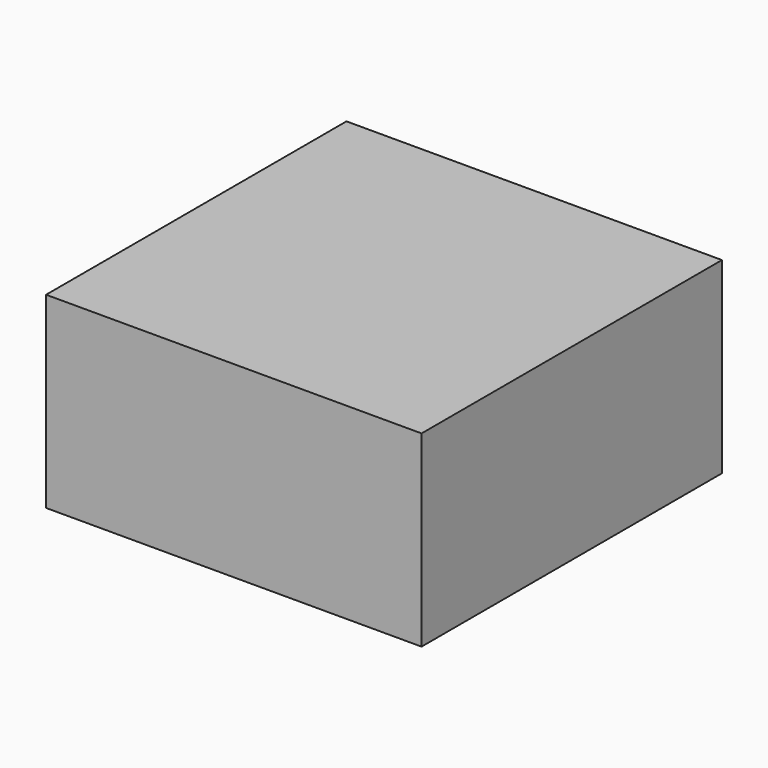
from build123d import *

# Parameters (mm, degrees)
F1_W     = 101.6
F1_H     = 101.6
F2_DEPTH = 101.6
F3_W     = 101.6
F3_H     = 101.6
F4_DEPTH = 101.6
F5_W     = 101.6
F5_H     = 101.6
F6_DEPTH = 101.6


# Not quite as in the source:
# - a variable given as a bare number and used for a length is read in inches; the dataset says mm whatever the document's units were


with BuildPart() as f2:
    # F1 (on Front) → F2 (new body, symmetric)
    with BuildSketch(Plane.XZ):
        Rectangle(F1_W, F1_H)
    extrude(amount=F2_DEPTH, both=True)

    # F3 (on face) → F4 (join)
    with BuildSketch(Plane.YZ.offset(50.8)):
        with Locations((50.8, 0)):
            Rectangle(F3_W, F3_H)
    extrude(amount=F4_DEPTH)

    # F5 (on face) → F6 (join)
    with BuildSketch(Plane.XZ):
        with Locations((101.6, 0)):
            Rectangle(F5_W, F5_H)
    extrude(amount=F6_DEPTH)


solid = f2.part
